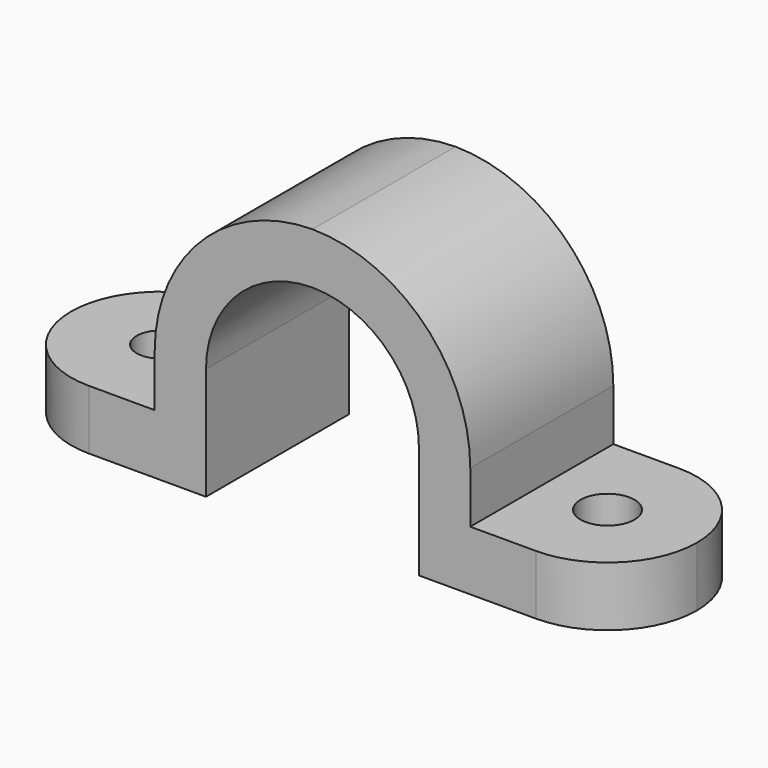
from build123d import *

# Parameters (mm, degrees)
F0_R        = 1.5930303601
F1_DEPTH    = 4
F0_R_2      = 1.8103813353
F0_W        = 18
F0_H        = 12
F0_W_2      = 1.5875
F2_DEPTH    = 18.1281324
F3_R        = 7.14375
F4_DEPTH    = 25.4
F5_W        = 14.2875
F5_H        = 12.0000014
F6_DEPTH    = 7.540625
F7_T1_DEPTH = 65.34


# Not quite as in the source:
# - a fillet or chamfer that OpenCascade refuses, or shapes differently, is made with other operations: its cross-section is extruded or revolved along the edge and cut away or added


with BuildPart() as f1:
    # F0 (on Top) → F1 (new body)
    with BuildSketch(Plane.XY):
        with BuildLine():
            ThreePointArc((0, 6), (1.7573593129, 1.7573593129), (6, 0))
            Line((6, 0), (10.4125, 0))
            Line((10.4125, 0), (10.4125, 12))
            Line((10.4125, 12), (6, 12))
            ThreePointArc((6, 12), (1.7573593129, 10.2426406871), (0, 6))
        make_face()
        with Locations((6, 6)):
            Circle(F0_R, mode=Mode.SUBTRACT)
    extrude(amount=F1_DEPTH)



with BuildPart() as f1b:
    # F0 (on Top) → F1, piece 2 (new body)
    with BuildSketch(Plane.XY):
        with BuildLine():
            Line((31.5875, 12), (31.5875, 0))
            Line((31.5875, 0), (36, 0))
            ThreePointArc((36, 0), (40.2426406871, 1.7573593129), (42, 6))
            ThreePointArc((42, 6), (40.2426406871, 10.2426406871), (36, 12))
            Line((36, 12), (31.5875, 12))
        make_face()
        with Locations((36, 6)):
            Circle(F0_R_2, mode=Mode.SUBTRACT)
    extrude(amount=F1_DEPTH)


with BuildPart() as f1_1:
    add(f1.part)

    add(f1b.part)  # F2 merges F1b
    # F0 (on Top) → F2 (join)
    with BuildSketch(Plane.XY):
        with Locations((21, 6)):
            Rectangle(F0_W, F0_H)
        with Locations((11.20625, 6)):
            Rectangle(F0_W_2, F0_H)
        with Locations((30.79375, 6)):
            Rectangle(F0_W_2, F0_H)
    extrude(amount=F2_DEPTH)

    # F3 (on face) → F4 (cut)
    with BuildSketch(Plane(origin=(0, 12, 0), x_dir=(-1, 0, 0), z_dir=(0, 1, 0))):
        with Locations((-20.9999947, 7.540625)):
            Circle(F3_R)
    extrude(amount=-F4_DEPTH, mode=Mode.SUBTRACT)

    # F5 (on face) → F6 (cut)
    with BuildSketch(Plane.XY):
        with Locations((20.9999947, 6.0000007)):
            Rectangle(F5_W, F5_H)
    extrude(amount=F6_DEPTH, mode=Mode.SUBTRACT)

    # F7: fillet of radius 10.668 on 2 edges, made by hand

    # F7_s2 → F7_t1 (cut)
    with BuildSketch(Plane.XZ.offset(-38.67)):
        with BuildLine():
            ThreePointArc((10.4125, 7.4601324), (13.5370848583, 15.0035475417), (21.0805, 18.1281324))
            Line((21.0805, 18.1281324), (10.4125, 18.1281324))
            Line((10.4125, 18.1281324), (10.4125, 7.4601324))
        make_face()
        with BuildLine():
            ThreePointArc((20.9195, 18.1281324), (28.4629151417, 15.0035475417), (31.5875, 7.4601324))
            Line((31.5875, 7.4601324), (31.5875, 18.1281324))
            Line((31.5875, 18.1281324), (20.9195, 18.1281324))
        make_face()
    extrude(amount=F7_T1_DEPTH, mode=Mode.SUBTRACT)


solid = f1_1.part
